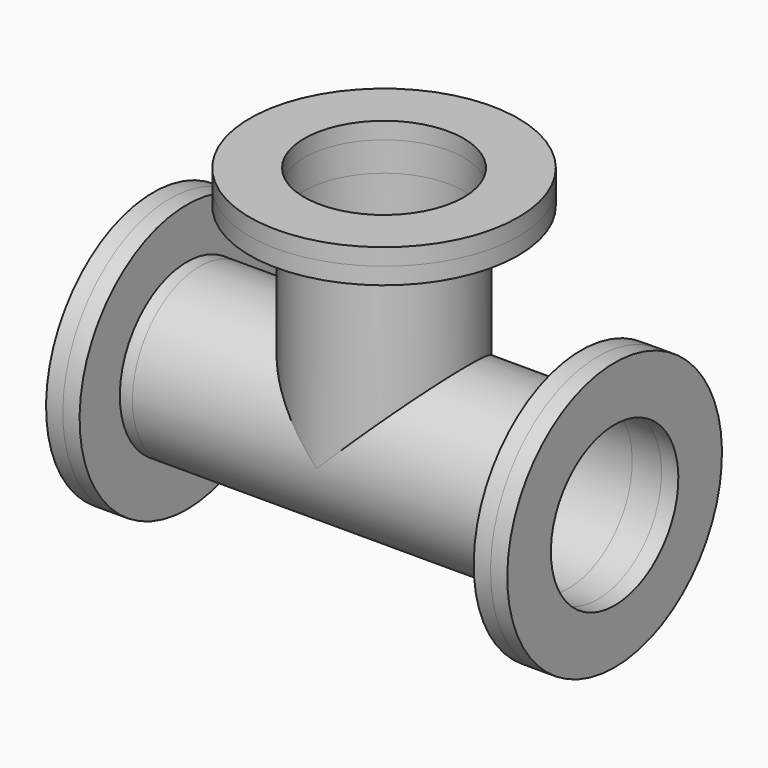
from build123d import *

# Parameters (mm, degrees)
F0_R      = 127
F0_R_2    = 120.65
F1_DEPTH  = 19.05
F2_R      = 203.2
F2_R_2    = 127
F2_R_3    = 120.65
F3_DEPTH  = 25.4
F9_ANGLE  = 90
F11_DEPTH = 558.8
F12_REACH = 841.8112448428
F13_DEPTH = 25.4
F14_DEPTH = 25.4
F15_DEPTH = 25.4


with BuildPart() as f1:
    # F0 (on Top) → F1 (new body)
    with BuildSketch(Plane.XY):
        Circle(F0_R)
        Circle(F0_R_2, mode=Mode.SUBTRACT)
    extrude(amount=F1_DEPTH)

    # F2 (on face) → F3 (join)
    with BuildSketch(Plane.XY.offset(19.05)):
        Circle(F2_R)
        Circle(F2_R_2, mode=Mode.SUBTRACT)
        Circle(F2_R_2)
        Circle(F2_R_3, mode=Mode.SUBTRACT)
    extrude(amount=F3_DEPTH)


with BuildPart() as f7_1:
    # F7: copy of F1
    add(f1.part.moved(Location((279.4, 0, -279.4))))


with BuildPart() as f7_1_1:
    # F9: moved
    add(f7_1.part.rotate(Axis((279.4, 122.1911609173, -279.4), (0, 1, 0)), F9_ANGLE))


with BuildPart() as f10_1:
    # F10: instance of F7_1
    add(f7_1_1.part.mirror(Plane.YZ))


with BuildPart() as f7_1_2:
    add(f7_1_1.part)

    # F11 (add, through all): a face of the model
    f11_faces = [f7_1_2.faces().sort_by_distance(p)[0] for p in [
        (279.4, 0, -155.9921024484),
    ]]

    add(f10_1.part)  # F11 merges F10_1
    extrude(f11_faces, amount=F11_DEPTH)


with BuildPart() as f1_1:
    add(f1.part)

    add(f7_1_2.part)  # F12 merges F7_1
    f12_end = f1_1.faces().sort_by_distance((0, 0, -152.4))[0]
    # F0 (on Top) → F12 (join, up to a face of the model that its end follows)
    with BuildSketch(Plane.XY):
        Circle(F0_R)
        Circle(F0_R_2, mode=Mode.SUBTRACT)
    f12_long = extrude(amount=-F12_REACH, mode=Mode.PRIVATE)
    add(split(f12_long, bisect_by=f12_end, keep=Keep.ALL, mode=Mode.PRIVATE).solids().sort_by_distance((-123.4078975516, 0, 0))[0])


with BuildPart() as f13:
    # F13 (new): a face of the model
    f13_faces = [f1_1.part.faces().sort_by_distance(p)[0] for p in [
        (323.85, 0, -81.9473639175),
    ]]
    extrude(f13_faces, amount=F13_DEPTH)


with BuildPart() as f14:
    # F14 (new): a face of the model
    f14_faces = [f1_1.part.faces().sort_by_distance(p)[0] for p in [
        (-323.85, 0, -81.9473639175),
    ]]
    extrude(f14_faces, amount=F14_DEPTH)


with BuildPart() as f15:
    # F15 (new): a face of the model
    f15_faces = [f1_1.part.faces().sort_by_distance(p)[0] for p in [
        (-197.4526360825, 0, 44.45),
    ]]
    extrude(f15_faces, amount=F15_DEPTH)


solid = Compound([f1_1.part, f13.part, f14.part, f15.part])
